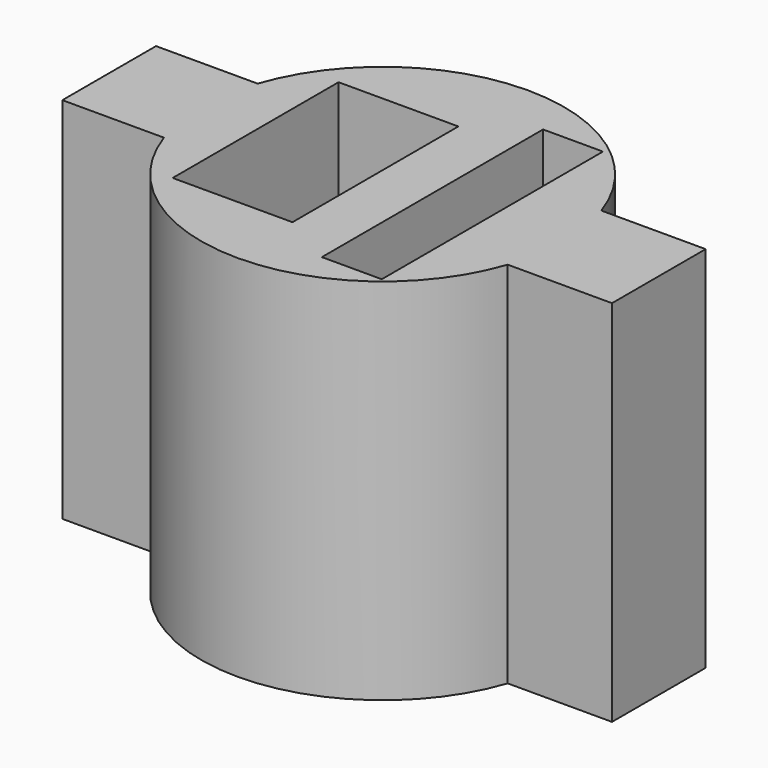
from build123d import *

# Parameters (mm, degrees)
F0_W     = 28.0003916717
F0_H     = 32.2663935487
F0_W_2   = 28.7430296161
F1_DEPTH = 101.6
F2_W     = 34.6587272506
F2_H     = 58.0717623234
F2_W_2   = 16.9384283945
F2_H_2   = 77.3962959647
F3_DEPTH = 12.7


# Not quite as in the source:
# - a feature names something its author has since deleted; it is built from what else it names


with BuildPart() as f1:
    # F0 (on Top) → F1 (new body)
    with BuildSketch(Plane.XY):
        with BuildLine():
            Line((-47.371, 16.1331967744), (-47.371, -16.1331967744))
            ThreePointArc((-47.371, -16.1331967744), (0, -50.0428983889), (47.371, -16.1331967744))
            Line((47.371, -16.1331967744), (47.371, 16.1331967744))
            ThreePointArc((47.371, 16.1331967744), (0, 50.0428983889), (-47.371, 16.1331967744))
        make_face()
        Polygon((-34.1799231236, -29.6225996721), (-34.1799231236, 27.5274003279), (-1.1599231236, 27.5274003279), (-1.1599231236, -29.6225996721), (-8.1120360752, -29.6225996721), align=None, mode=Mode.SUBTRACT)
        Polygon((13.945407662, -38.3726616568), (13.945407662, 37.8273383432), (30.455407662, 37.8273383432), (30.455407662, -38.3726616568), (18.8453282475, -38.3726616568), align=None, mode=Mode.SUBTRACT)
        with Locations((-61.3711958359, 0)):
            Rectangle(F0_W, F0_H)
        with Locations((61.7425148081, 0)):
            Rectangle(F0_W_2, F0_H)
    extrude(amount=F1_DEPTH)

    # F2 (on Top) → F3 (join)
    with BuildSketch(Plane.XY):
        with Locations((-17.2371207664, -0.9217876941)):
            Rectangle(F2_W, F2_H)
        with Locations((22.572400514, -0.1084208488)):
            Rectangle(F2_W_2, F2_H_2)
    extrude(amount=F3_DEPTH)


solid = f1.part
